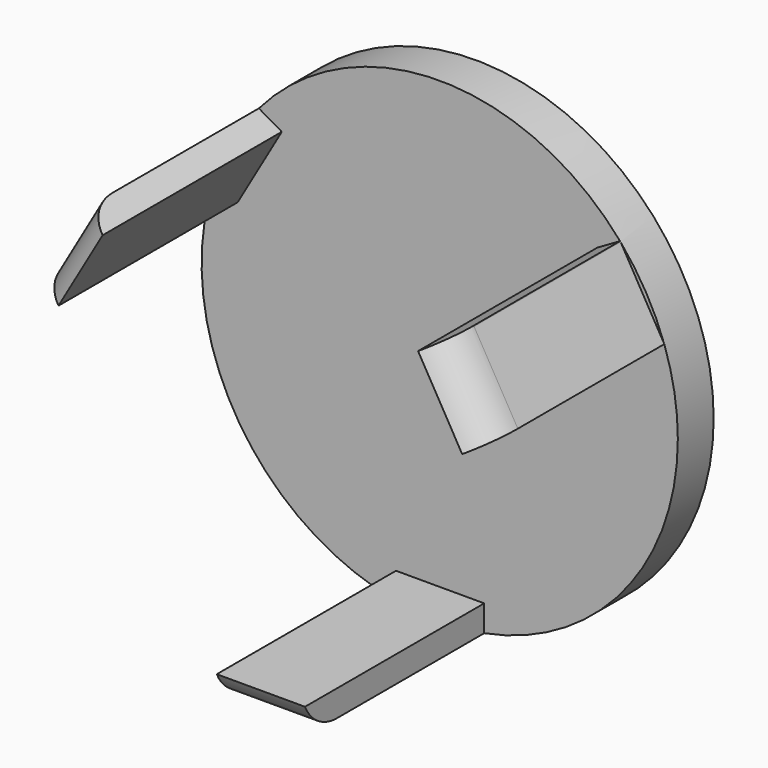
from build123d import *

# Parameters (mm, degrees)
F0_R        = 27
F1_DEPTH    = 5.08
F3_DEPTH    = 25.4
F4_T1_DEPTH = 33.0899649141
F4_T3_DEPTH = 33.0899649141
F4_T5_DEPTH = 33.0899649141


# Not quite as in the source:
# - a fillet or chamfer that OpenCascade refuses, or shapes differently, is made with other operations: its cross-section is extruded or revolved along the edge and cut away or added


with BuildPart() as f1:
    # F0 (on Front) → F1 (new body)
    with BuildSketch(Plane.XZ):
        Circle(F0_R)
    extrude(amount=F1_DEPTH)

    # F2 (on face) → F3 (join)
    with BuildSketch(Plane.XZ.offset(5.08)):
        with BuildLine():
            ThreePointArc((-25.4641942221, 8.9763473985), (-25.4782526607, 8.9363662278), (-25.4922483252, 8.8963630393))
            Line((-25.4922483252, 8.8963630393), (-22.90776578, 7.4042113462))
            Line((-22.90776578, 7.4042113462), (-17.90776578, 16.064465384))
            Line((-17.90776578, 16.064465384), (-20.5058419913, 17.564465384))
            Line((-20.5058419913, 17.564465384), (-25.4641942221, 8.9763473985))
        make_face()
        with BuildLine():
            Line((22.8661180108, 7.4763473985), (25.4641942221, 8.9763473985))
            Line((25.4641942221, 8.9763473985), (20.5058419913, 17.564465384))
            ThreePointArc((20.5058419913, 17.564465384), (20.4782465011, 17.5966309343), (20.4506005559, 17.6287531295))
            Line((20.4506005559, 17.6287531295), (17.8661180108, 16.1366014363))
            Line((17.8661180108, 16.1366014363), (22.8661180108, 7.4763473985))
        make_face()
        with BuildLine():
            Line((-4.9583522308, -23.5408127825), (-4.9583522308, -26.5408127825))
            Line((-4.9583522308, -26.5408127825), (4.9583522308, -26.5408127825))
            ThreePointArc((4.9583522308, -26.5408127825), (5.0000061596, -26.5329971621), (5.0416477692, -26.5251161689))
            Line((5.0416477692, -26.5251161689), (5.0416477692, -23.5408127825))
            Line((5.0416477692, -23.5408127825), (-4.9583522308, -23.5408127825))
        make_face()
    extrude(amount=F3_DEPTH)

    # F4: fillet of radius 5.08 on 3 edges, made by hand

    # F4_s2 → F4_t1 (cut)
    with BuildSketch(Plane(origin=(8.2724912285, 0, 14.328375113), x_dir=(0, 1, 0), z_dir=(-0.5, 0, -0.8660254038))):
        with BuildLine():
            ThreePointArc((-25.8453479095, -26.5408127825), (-28.6057826579, -25.7253643416), (-30.48, -23.5408127825))
            Line((-30.48, -23.5408127825), (-30.48, -26.5408127825))
            Line((-30.48, -26.5408127825), (-25.8453479095, -26.5408127825))
        make_face()
    extrude(amount=F4_T1_DEPTH, mode=Mode.SUBTRACT)

    # F4_s4 → F4_t3 (cut)
    with BuildSketch(Plane.YZ.offset(-16.544982457)):
        with BuildLine():
            ThreePointArc((-25.8453479095, -26.5408127825), (-28.6057826579, -25.7253643416), (-30.48, -23.5408127825))
            Line((-30.48, -23.5408127825), (-30.48, -26.5408127825))
            Line((-30.48, -26.5408127825), (-25.8453479095, -26.5408127825))
        make_face()
    extrude(amount=F4_T3_DEPTH, mode=Mode.SUBTRACT)

    # F4_s6 → F4_t5 (cut)
    with BuildSketch(Plane(origin=(8.2724912285, 0, -14.328375113), x_dir=(0, 1, 0), z_dir=(-0.5, 0, 0.8660254038))):
        with BuildLine():
            ThreePointArc((-25.8453479095, -26.5408127825), (-28.6057826579, -25.7253643416), (-30.48, -23.5408127825))
            Line((-30.48, -23.5408127825), (-30.48, -26.5408127825))
            Line((-30.48, -26.5408127825), (-25.8453479095, -26.5408127825))
        make_face()
    extrude(amount=F4_T5_DEPTH, mode=Mode.SUBTRACT)


solid = f1.part
